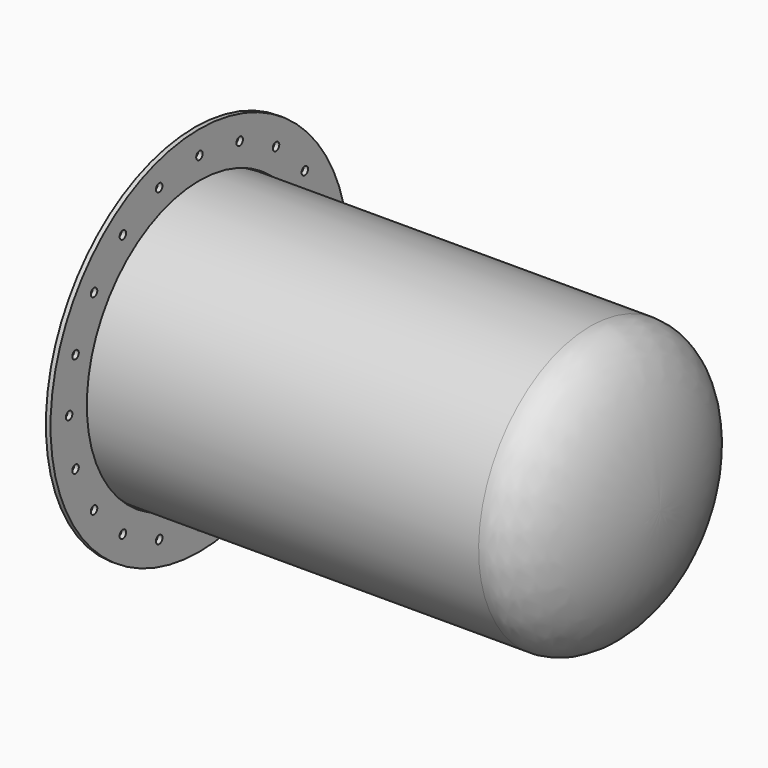
from build123d import *

# Parameters (mm, degrees)
F2_T            = -2.5
F3_W            = 10
F3_H            = 97.5
F6_D            = 17.5
F6_COPIES_COUNT = 20


# Not quite as in the source:
# - a pattern or mirror of a feature is missing from the dataset's text; its kind, count and spacing are read off the source's solid


with BuildPart() as f1:
    # F0 (on Front) → F1 (revolve)
    with BuildSketch(Plane.XZ):
        with BuildLine():
            Line((0, 300), (0, 0))
            Line((0, 0), (1000, 0))
            add(Edge.make_bspline(
                [(1000, 0), (1000, 300), (850, 300)],
                knots=[4.7123889804, 4.7123889804, 4.7123889804, 6.2831853072, 6.2831853072, 6.2831853072], degree=2, weights=[1, 0.7071067812, 1]))
            Line((850, 300), (0, 300))
        make_face()
    revolve(axis=Axis((-240.407243371, 0, 0), (-1, 0, 0)))

    # F2
    f2_openings = [f1.faces().sort_by_distance(p)[0] for p in [
        (0, 0, 0),
    ]]
    offset(amount=F2_T, openings=f2_openings)


with BuildPart() as f4:
    # F3 (on Front) → F4 (revolve)
    with BuildSketch(Plane.XZ):
        with Locations((5, 351.25)):
            Rectangle(F3_W, F3_H)
    revolve(axis=Axis((-40.1947914194, 0, 0), (-1, 0, 0)))

    # F6 (through all)
    with Locations(Plane(origin=(0, 0, 0), x_dir=(0, -1, 0), z_dir=(-1, 0, 0))):
        with Locations((0, 350)):
            f6 = Hole(F6_D / 2)

    # F6_copies: F6 ×20 about axis
    f6_copies_axis = Axis((0, 0, 0), (1, 0, 0))
    for i in range(1, F6_COPIES_COUNT):
        add(f6.rotate(f6_copies_axis, i * 360 / F6_COPIES_COUNT), mode=Mode.SUBTRACT)


solid = Compound([f1.part, f4.part])
